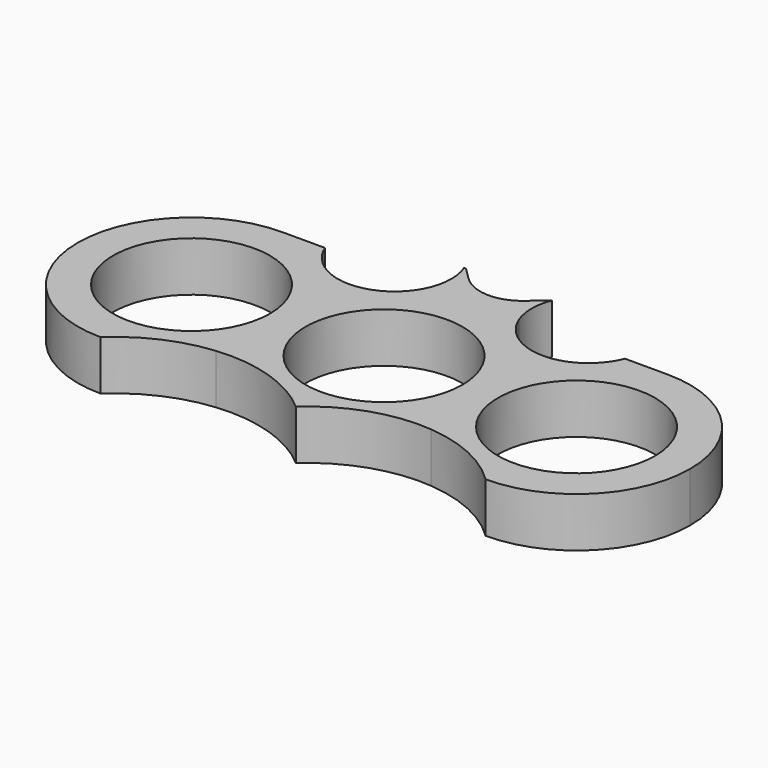
from build123d import *

# Parameters (mm, degrees)
F0_R     = 11.05
F1_DEPTH = 7


# Not quite as in the source:
# - a feature names something its author has since deleted; it is built from what else it names


with BuildPart() as f1:
    # F0 (on Top) → F1 (new body)
    with BuildSketch(Plane.XY):
        with BuildLine():
            ThreePointArc((-19.2783924252, 3.2977389637), (-20.321649546, -2.3852041509), (-23.3153727308, -7.3270509067))
            ThreePointArc((-23.3153727308, -7.3270509067), (-15.247882117, -8.2153155431), (-8.1783924252, -12.2022610363))
            ThreePointArc((-8.1783924252, -12.2022610363), (-1.221278488, -8.1070481694), (6.7932734583, -7.1379455637))
            ThreePointArc((6.7932734583, -7.1379455637), (2.9292273158, 3.7914733565), (7.4601219716, 14.4617144101))
            ThreePointArc((7.4601219716, 14.4617144101), (1.8212672524, 15.0889872554), (-1.9835406039, 19.2977389637))
            Line((-1.9835406039, 19.2977389637), (-14.3732442464, 19.2977389637))
            ThreePointArc((-14.3732442464, 19.2977389637), (-18.1780521028, 15.0889872554), (-23.816906822, 14.4617144101))
            ThreePointArc((-23.816906822, 14.4617144101), (-20.4563856506, 9.3233605229), (-19.2783924252, 3.2977389637))
        make_face()
        with Locations((-8.1783924252, 3.2977389637)):
            Circle(F0_R, mode=Mode.SUBTRACT)
        with BuildLine():
            ThreePointArc((-28.490516072, 17.7865185747), (-31.8013587595, 18.915364804), (-35.2783924252, 19.2977389637))
            ThreePointArc((-35.2783924252, 19.2977389637), (-51.2783924252, 3.2977389637), (-35.2783924252, -12.7022610363))
            ThreePointArc((-35.2783924252, -12.7022610363), (-29.74444778, -9.0185588521), (-23.3153727308, -7.3270509067))
            ThreePointArc((-23.3153727308, -7.3270509067), (-20.321649546, -2.3852041509), (-19.2783924252, 3.2977389637))
            ThreePointArc((-19.2783924252, 3.2977389637), (-20.4563856506, 9.3233605229), (-23.816906822, 14.4617144101))
            ThreePointArc((-23.816906822, 14.4617144101), (-26.4619172405, 15.6908779087), (-28.490516072, 17.7865185747))
        make_face()
        with Locations((-35.2783924252, 3.2977389637)):
            Circle(F0_R, mode=Mode.SUBTRACT)
        with BuildLine():
            ThreePointArc((7.4601219716, 14.4617144101), (2.9292273158, 3.7914733565), (6.7932734583, -7.1379455637))
            ThreePointArc((6.7932734583, -7.1379455637), (13.3416443494, -8.8647019853), (18.9216075748, -12.7022610363))
            ThreePointArc((18.9216075748, -12.7022610363), (30.2353160738, -8.0159695352), (34.9216075748, 3.2977389637))
            ThreePointArc((34.9216075748, 3.2977389637), (30.2353160738, 14.6114474627), (18.9216075748, 19.2977389637))
            ThreePointArc((18.9216075748, 19.2977389637), (15.4445739091, 18.915364804), (12.1337312216, 17.7865185747))
            ThreePointArc((12.1337312216, 17.7865185747), (10.1051323901, 15.6908779087), (7.4601219716, 14.4617144101))
        make_face()
        with Locations((18.9216075748, 3.2977389637)):
            Circle(F0_R, mode=Mode.SUBTRACT)
        with BuildLine():
            Line((-29.2757110635, 19.2977389637), (-35.2783924252, 19.2977389637))
            ThreePointArc((-35.2783924252, 19.2977389637), (-31.8013587595, 18.915364804), (-28.490516072, 17.7865185747))
            ThreePointArc((-28.490516072, 17.7865185747), (-28.923441503, 18.5211753113), (-29.2757110635, 19.2977389637))
        make_face()
        with BuildLine():
            Line((18.9216075748, 19.2977389637), (12.9189262131, 19.2977389637))
            ThreePointArc((12.9189262131, 19.2977389637), (12.5666566526, 18.5211753113), (12.1337312216, 17.7865185747))
            ThreePointArc((12.1337312216, 17.7865185747), (15.4445739091, 18.915364804), (18.9216075748, 19.2977389637))
        make_face()
        with BuildLine():
            ThreePointArc((-13.824477655, 22.2096319377), (-13.9628662658, 20.7280563015), (-14.3732442464, 19.2977389637))
            Line((-14.3732442464, 19.2977389637), (-1.9835406039, 19.2977389637))
            ThreePointArc((-1.9835406039, 19.2977389637), (-2.5323071954, 22.2096319377), (-1.9835406039, 25.1215249117))
            Line((-1.9835406039, 25.1215249117), (-3.9835406039, 23.4114221363))
            ThreePointArc((-3.9835406039, 23.4114221363), (-8.1817639697, 21.709585029), (-12.3732442464, 23.4279627693))
            Line((-12.3732442464, 23.4279627693), (-14.0983548132, 25.1215249117))
            Line((-14.0983548132, 25.1215249117), (-14.3732442464, 25.1215249117))
            ThreePointArc((-14.3732442464, 25.1215249117), (-13.9628662658, 23.691207574), (-13.824477655, 22.2096319377))
        make_face()
    extrude(amount=F1_DEPTH)


solid = f1.part
